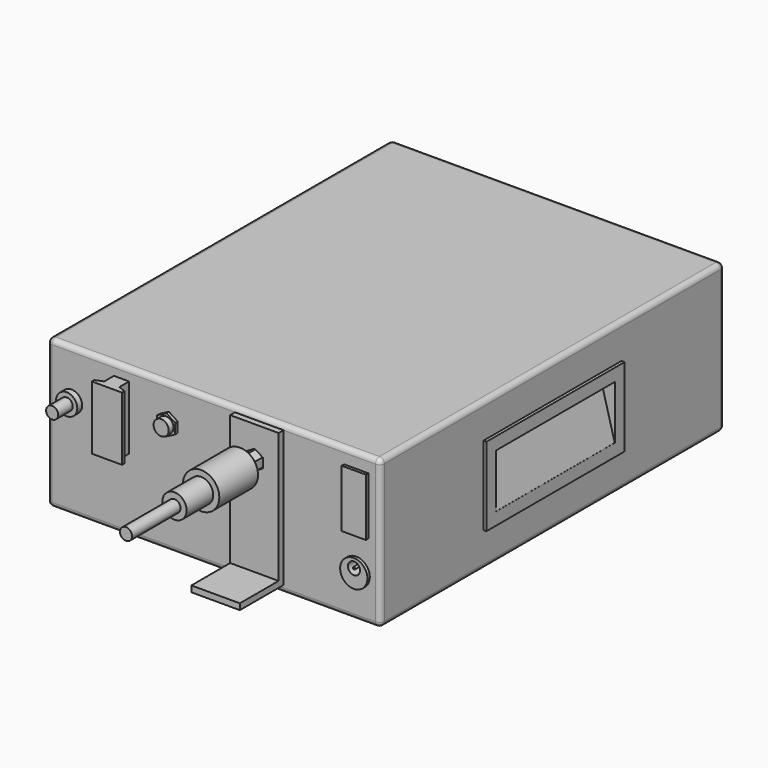
from build123d import *

# Parameters (mm, degrees)
F0_W       = 174.625
F0_H       = 77.7875
F1_DEPTH   = 225.425
F2_W       = 90.4875
F2_H       = 41.275
F3_DEPTH   = 1.5875
F4_W       = 90.4875
F4_H       = 41.275
F5_DEPTH   = 1.5875
F6_R       = 2.54
F9_W       = 77.7875
F9_H       = 27.5794637142
F10_DEPTH  = 25.4
F13_W      = 77.7875
F13_H      = 27.1685884801
F14_DEPTH  = 25.4
F15_R      = 7.14375
F16_DEPTH  = 1.5875
F17_R      = 3.175
F18_DEPTH  = 12.7
F19_R      = 0.635
F20_DEPTH  = 12.7
F21_W      = 12.7
F21_H      = 30.1625
F22_DEPTH  = 1.5875
F24_DEPTH  = 12.7
F25_R      = 9.525
F26_DEPTH  = 25.4
F27_R      = 6.35
F28_DEPTH  = 17.4625
F29_R      = 3.175
F30_DEPTH  = 31.75
F32_DEPTH  = 1.5875
F33_R      = 3.96875
F34_DEPTH  = 3.175
F35_W      = 7.9375
F35_H      = 33.3375
F36_DEPTH  = 6.35
F36_FACE_W = 7.9375
F36_FACE_H = 33.3375
F38_W      = 15.875
F38_H      = 33.3375
F40_W      = 15.875
F40_H      = 33.3375
F41_DEPTH  = 1.5875
F42_R      = 5.55625
F43_DEPTH  = 3.175
F44_R      = 3.175
F45_DEPTH  = 9.525
F46_W      = 25.4
F46_H      = 71.4375
F47_DEPTH  = 3.175
F49_DEPTH  = 228.601
F50_W      = 25.4
F50_H      = 3.175
F51_DEPTH  = 25.4


with BuildPart() as f1:
    # F0 (on Front) → F1 (new body)
    with BuildSketch(Plane.XZ):
        Rectangle(F0_W, F0_H)
    extrude(amount=F1_DEPTH)

    # F2 (on face) → F3 (join)
    with BuildSketch(Plane(origin=(-87.3125, 0, 0), x_dir=(0, -1, 0), z_dir=(-1, 0, 0))):
        with Locations((112.7125, 0)):
            Rectangle(F2_W, F2_H)
    extrude(amount=F3_DEPTH)

    # F4 (on face) → F5 (join)
    with BuildSketch(Plane.YZ.offset(87.3125)):
        with Locations((-112.7125, 0)):
            Rectangle(F4_W, F4_H)
    extrude(amount=F5_DEPTH)

    # F6
    f6_edges = [f1.edges().sort_by_distance(p)[0] for p in [
        (0, 0, 38.89375),
        (87.3125, 0, 0),
        (87.3125, -112.7125, 38.89375),
        (87.3125, -112.7125, -38.89375),
        (-87.3125, -112.7125, 38.89375),
        (0, -225.425, 38.89375),
        (87.3125, -225.425, 0),
        (-87.3125, -225.425, 0),
        (0, -225.425, -38.89375),
        (-87.3125, -112.7125, -38.89375),
        (0, 0, -38.89375),
        (-87.3125, 0, 0),
    ]]
    fillet(f6_edges, radius=F6_R)

    # F9 (on face) → F10 (cut)
    with BuildSketch(Plane(origin=(-79.3729541982, 0, 21.2679189783), x_dir=(0, 1, 0), z_dir=(0.9659258263, 0, -0.2588190451))):
        with Locations((-112.7125, -22.8035754926)):
            Rectangle(F9_W, F9_H)
    extrude(amount=-F10_DEPTH, mode=Mode.SUBTRACT)

    # F13 (on face) → F14 (cut)
    with BuildSketch(Plane(origin=(79.3729541982, 0, 21.2679189783), x_dir=(0, -1, 0), z_dir=(-0.9659258263, 0, -0.2588190451))):
        with Locations((112.7125, -23.0090131096)):
            Rectangle(F13_W, F13_H)
    extrude(amount=-F14_DEPTH, mode=Mode.SUBTRACT)

    # F15 (on face) → F16 (join)
    with BuildSketch(Plane.XZ.offset(225.425)):
        with Locations((74.6125, -16.66875)):
            Circle(F15_R)
    extrude(amount=F16_DEPTH)

    # F17 (on face) → F18 (cut)
    with BuildSketch(Plane.XZ.offset(227.0125)):
        with Locations((74.7314542532, -14.2884904529)):
            Circle(F17_R)
    extrude(amount=-F18_DEPTH, mode=Mode.SUBTRACT)

    # F19 (on face) → F20 (join)
    with BuildSketch(Plane.XZ.offset(214.3125)):
        with Locations((74.7314542532, -14.2884904529)):
            Circle(F19_R)
    extrude(amount=F20_DEPTH)

    # F21 (on face) → F22 (join)
    with BuildSketch(Plane.XZ.offset(225.425)):
        with Locations((74.6125, 15.875)):
            Rectangle(F21_W, F21_H)
    extrude(amount=F22_DEPTH)

    # F23 (on face) → F24 (join)
    with BuildSketch(Plane.XZ.offset(225.425)):
        Polygon((23.839955207, 15.2611144816), (27.7949063788, 17.5762091475), (27.7674511717, 22.158844666), (23.785044793, 24.4263855184), (19.8300936212, 22.1112908525), (19.8575488283, 17.528655334), align=None)
    extrude(amount=F24_DEPTH)

    # F31 (on face) → F32 (join)
    with BuildSketch(Plane.XZ.offset(225.425)):
        Polygon((-24.0715896818, 14.350595393), (-19.1848334043, 16.8727944502), (-18.9257437225, 22.3659490572), (-23.5534103182, 25.336904607), (-28.4401665957, 22.8147055498), (-28.6992562775, 17.3215509428), align=None)
    extrude(amount=F32_DEPTH)

    # F33 (on face) → F34 (join)
    with BuildSketch(Plane.XZ.offset(227.0125)):
        with Locations((-23.8125, 19.84375)):
            Circle(F33_R)
    extrude(amount=F34_DEPTH)

    # F35 (on face) → F36 (join)
    with BuildSketch(Plane.XZ.offset(225.425)):
        with Locations((-48.41875, 15.875)):
            Rectangle(F35_W, F35_H)
    extrude(amount=F36_DEPTH)

    # F36_face (on face) → F39 section 0
    with BuildSketch(Plane(origin=(-48.41875, -231.775, 15.875), x_dir=(1, 0, 0), z_dir=(0, -1, 0))):
        Rectangle(F36_FACE_W, F36_FACE_H)
    # F38 (on offset) → F39 section 1
    with BuildSketch(Plane.XZ.offset(233.3625)):
        with Locations((-48.41875, 15.875)):
            Rectangle(F38_W, F38_H)
    loft()

    # F40 (on face) → F41 (join)
    with BuildSketch(Plane.XZ.offset(233.3625)):
        with Locations((-48.41875, 15.875)):
            Rectangle(F40_W, F40_H)
    extrude(amount=F41_DEPTH)

    # F42 (on face) → F43 (join)
    with BuildSketch(Plane.XZ.offset(225.425)):
        with Locations((-74.6125, 13.49375)):
            Circle(F42_R)
    extrude(amount=F43_DEPTH)

    # F44 (on face) → F45 (join)
    with BuildSketch(Plane.XZ.offset(228.6)):
        with Locations((-74.6125, 13.49375)):
            Circle(F44_R)
    extrude(amount=F45_DEPTH)


with BuildPart() as f26:
    # F25 (on face) → F26 (new body)
    with BuildSketch(Plane.XZ.offset(238.125)):
        with Locations((23.8125, 19.84375)):
            Circle(F25_R)
    extrude(amount=F26_DEPTH)


with BuildPart() as f28:
    # F27 (on face) → F28 (new body)
    with BuildSketch(Plane.XZ.offset(263.525)):
        with Locations((23.8125, 19.84375)):
            Circle(F27_R)
    extrude(amount=F28_DEPTH)


with BuildPart() as f30:
    # F29 (on face) → F30 (new body)
    with BuildSketch(Plane.XZ.offset(280.9875)):
        with Locations((23.8125, 19.84375)):
            Circle(F29_R)
    extrude(amount=F30_DEPTH)


with BuildPart() as f47:
    # F46 (on face) → F47 (new body)
    with BuildSketch(Plane.XZ.offset(225.425)):
        with Locations((23.785044793, 0.635)):
            Rectangle(F46_W, F46_H)
    extrude(amount=F47_DEPTH)

    # F48 (on face) → F49 (cut, through all)
    with BuildSketch(Plane.XZ.offset(228.6)):
        Polygon((23.785044793, 14.7111061069), (28.230044793, 17.2774280535), (28.230044793, 22.4100719465), (23.785044793, 24.9763938931), (19.340044793, 22.4100719465), (19.340044793, 17.2774280535), align=None)
    extrude(amount=-F49_DEPTH, mode=Mode.SUBTRACT)

    # F50 (on face) → F51 (join)
    with BuildSketch(Plane.XZ.offset(228.6)):
        with Locations((23.785044793, -33.49625)):
            Rectangle(F50_W, F50_H)
    extrude(amount=F51_DEPTH)


solid = Compound([f1.part, f26.part, f28.part, f30.part, f47.part])
